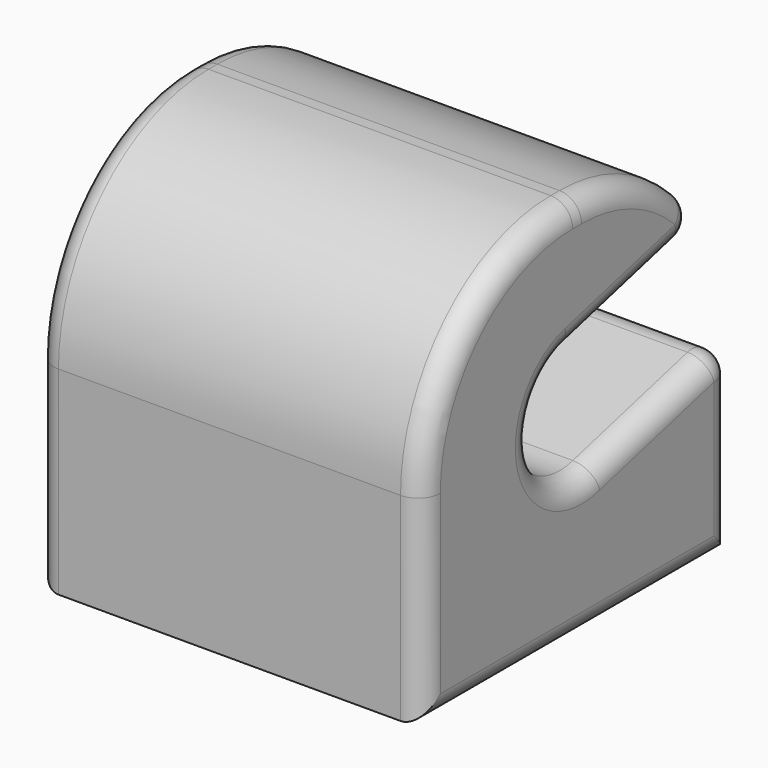
from build123d import *

# Parameters (mm, degrees)
F0_W     = 35
F0_H     = 35
F1_DEPTH = 35
F2_R     = 17
F5_DEPTH = 35.001
F6_R     = 2


with BuildPart() as f1:
    # F0 (on Top) → F1 (new body)
    with BuildSketch(Plane.XY):
        Rectangle(F0_W, F0_H)
    extrude(amount=F1_DEPTH)

    # F2
    f2_edges = [f1.edges().sort_by_distance(p)[0] for p in [
        (0, -17.5, 35),
        (0, 17.5, 35),
    ]]
    fillet(f2_edges, radius=F2_R)

    # F4 (on face) → F5 (cut, through all)
    with BuildSketch(Plane.YZ.offset(17.5)):
        with BuildLine():
            ThreePointArc((17.5, 18), (16.7637891964, 22.9486524402), (14.6189222384, 27.4686870699))
            Line((14.6189222384, 27.4686870699), (-0.8730111465, 23.4686870699))
            ThreePointArc((-0.8730111465, 23.4686870699), (-4.8066349175, 16.7018804151), (2.0080666152, 12.8518270003))
            Line((2.0080666152, 12.8518270003), (17.5, 16.8518270003))
            Line((17.5, 16.8518270003), (17.5, 18))
        make_face()
    extrude(amount=-F5_DEPTH, mode=Mode.SUBTRACT)

    # F6
    f6_edges = [f1.edges().sort_by_distance(p)[0] for p in [
        (17.5, -17.5, 9),
        (17.5, 0, 0),
        (17.5, 17.5, 8.425914),
        (17.5, 9.754033, 14.851827),
        (17.5, -4.806635, 16.70188),
        (17.5, 6.872956, 25.468687),
        (17.5, 8.50101, 32.999461),
        (17.5, 0, 35),
        (17.5, -12.520815, 30.020815),
        (-17.5, 0, 0),
        (-17.5, -17.5, 9),
        (-17.5, -12.520815, 30.020815),
        (-17.5, 0, 35),
        (-17.5, 8.50101, 32.999461),
        (-17.5, 6.872956, 25.468687),
        (-17.5, -4.806635, 16.70188),
        (-17.5, 9.754033, 14.851827),
        (-17.5, 17.5, 8.425914),
        (0, 17.5, 16.851827),
        (0, 14.618922, 27.468687),
    ]]
    fillet(f6_edges, radius=F6_R)


solid = f1.part
